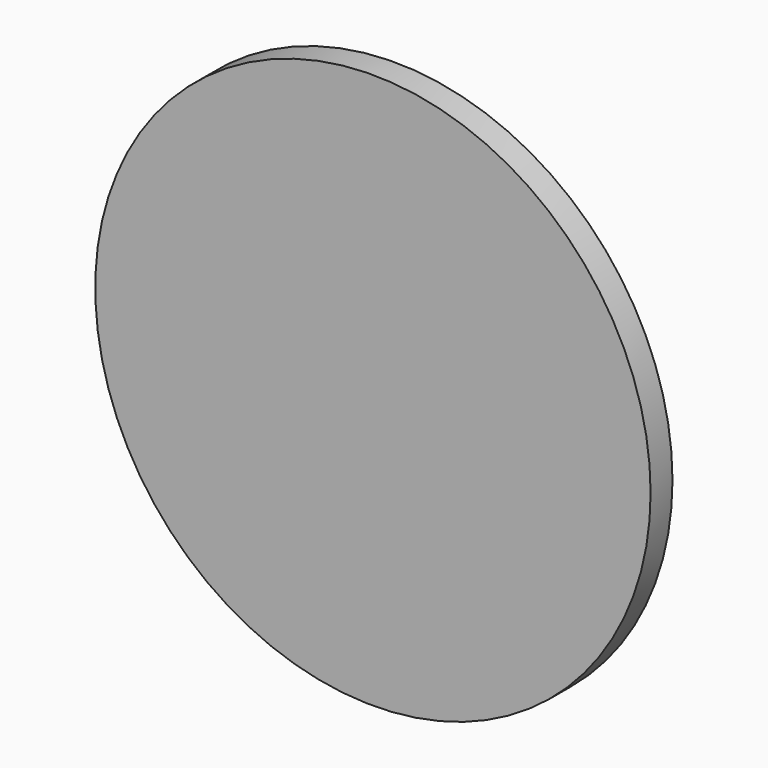
from build123d import *

# Parameters (mm, degrees)
F1_R     = 101.5
F3_DEPTH = 10


# Not quite as in the source:
# - the program builds the solid bodies; features that only make, move or delete a surface that nothing else refers to are left out


with BuildPart() as f3:
    # F1 (on face) → F3 (new body)
    with BuildSketch(Plane.XZ):
        Circle(F1_R)
    extrude(amount=F3_DEPTH)


solid = f3.part
